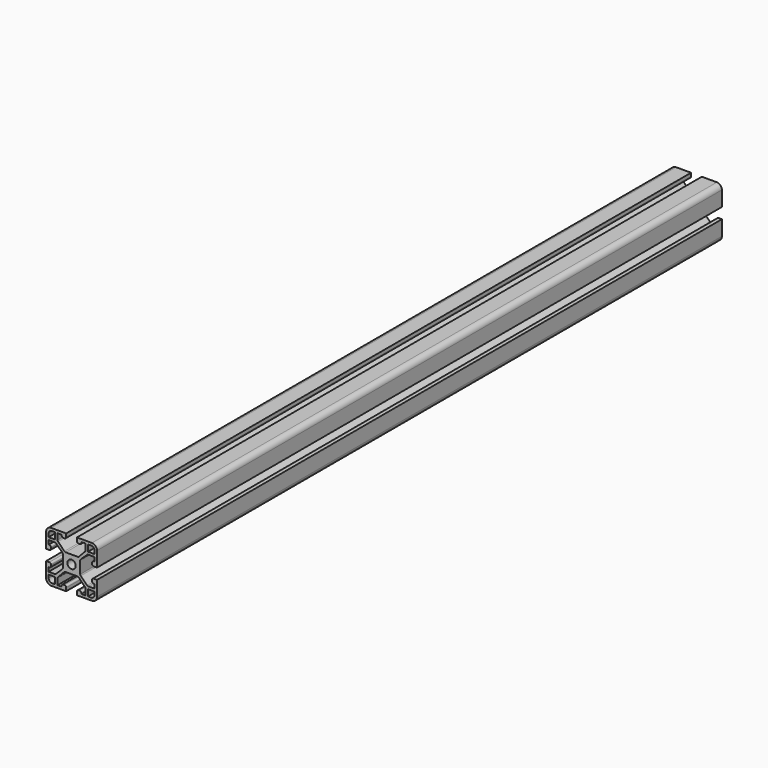
from build123d import *

# Parameters (mm, degrees)
F0_R     = 2.45
F1_DEPTH = 460


# Not quite as in the source:
# - ends of sketch curves that miss each other by under 0.0002 mm in the source are joined


with BuildPart() as f1:
    # F0 (on Front) → F1 (new body)
    with BuildSketch(Plane.XZ):
        with BuildLine():
            Line((-3.1749674082, 15), (-12, 15))
            ThreePointArc((-12, 15), (-14.1213203436, 14.1213203436), (-15, 12))
            Line((-15, 12), (-15, 3.175))
            Line((-15, 3.175), (-13.0855346263, 3.175))
            ThreePointArc((-13.0855346263, 3.175), (-12.3835980145, 3.4627605788), (-12.0856407741, 4.1604300138))
            Line((-12.0856407741, 4.1604300138), (-12.0761692778, 4.8104300138))
            ThreePointArc((-12.0761692778, 4.8104300138), (-12.3638237087, 5.5269366118), (-13.0760631299, 5.825))
            Line((-13.0760631299, 5.825), (-13.5, 5.825))
            Line((-13.5, 5.825), (-13.5, 8.225))
            Line((-13.5, 8.225), (-9.8968845016, 8.225))
            ThreePointArc((-9.8968845016, 8.225), (-9.5279915195, 8.1544718757), (-9.2111331975, 7.9528359354))
            Line((-9.2111331975, 7.9528359354), (-5.4142486959, 4.3754933338))
            ThreePointArc((-5.4142486959, 4.3754933338), (-5.1819174045, 4.0440465354), (-5.1, 3.6476573984))
            Line((-5.1, 3.6476573984), (-5.1, -3.4999243287))
            ThreePointArc((-5.1, -3.4999243287), (-5.1782354607, -3.8876744211), (-5.4007002683, -4.2147528992))
            Line((-5.4007002683, -4.2147528992), (-9.2084959767, -7.9398285705))
            ThreePointArc((-9.2084959767, -7.9398285705), (-9.5301904718, -8.1509666761), (-9.9077957084, -8.225))
            Line((-9.9077957084, -8.225), (-13.5, -8.225))
            Line((-13.5, -8.225), (-13.5, -5.825))
            Line((-13.5, -5.825), (-13.0760631299, -5.825))
            ThreePointArc((-13.0760631299, -5.825), (-12.3638237087, -5.5269366118), (-12.0761692778, -4.8104300138))
            Line((-12.0761692778, -4.8104300138), (-12.0856407741, -4.1604300138))
            ThreePointArc((-12.0856407741, -4.1604300138), (-12.3835980145, -3.4627605788), (-13.0855346263, -3.175))
            Line((-13.0855346263, -3.175), (-15, -3.175))
            Line((-15, -3.175), (-15, -12))
            ThreePointArc((-15, -12), (-14.1213203436, -14.1213203436), (-12, -15))
            Line((-12, -15), (-3.175, -15))
            Line((-3.175, -15), (-3.175, -13.0855346263))
            ThreePointArc((-3.175, -13.0855346263), (-3.4627605788, -12.3835980145), (-4.1604300138, -12.0856407741))
            Line((-4.1604300138, -12.0856407741), (-4.8104300138, -12.0761692778))
            ThreePointArc((-4.8104300138, -12.0761692778), (-5.5269366118, -12.3638237087), (-5.825, -13.0760631299))
            Line((-5.825, -13.0760631299), (-5.825, -13.5))
            Line((-5.825, -13.5), (-8.225, -13.5))
            Line((-8.225, -13.5), (-8.225, -9.8968845016))
            ThreePointArc((-8.225, -9.8968845016), (-8.1544718757, -9.5279915195), (-7.9528359354, -9.2111331975))
            Line((-7.9528359354, -9.2111331975), (-4.3754933338, -5.4142486959))
            ThreePointArc((-4.3754933338, -5.4142486959), (-4.0440465354, -5.1819174045), (-3.6476573984, -5.1))
            Line((-3.6476573984, -5.1), (3.4999243287, -5.1))
            ThreePointArc((3.4999243287, -5.1), (3.8876744211, -5.1782354607), (4.2147528992, -5.4007002683))
            Line((4.2147528992, -5.4007002683), (7.9398285705, -9.2084959767))
            ThreePointArc((7.9398285705, -9.2084959767), (8.1509666761, -9.5301904718), (8.225, -9.9077957084))
            Line((8.225, -9.9077957084), (8.225, -13.5))
            Line((8.225, -13.5), (5.825, -13.5))
            Line((5.825, -13.5), (5.825, -13.0760631299))
            ThreePointArc((5.825, -13.0760631299), (5.5269366118, -12.3638237087), (4.8104300138, -12.0761692778))
            Line((4.8104300138, -12.0761692778), (4.1604300138, -12.0856407741))
            ThreePointArc((4.1604300138, -12.0856407741), (3.4627605788, -12.3835980145), (3.175, -13.0855346263))
            Line((3.175, -13.0855346263), (3.175, -15))
            Line((3.175, -15), (12, -15))
            ThreePointArc((12, -15), (14.1213203436, -14.1213203436), (15, -12))
            Line((15, -12), (15, -3.175))
            Line((15, -3.175), (13.0855346263, -3.175))
            ThreePointArc((13.0855346263, -3.175), (12.3835980145, -3.4627605788), (12.0856407741, -4.1604300138))
            Line((12.0856407741, -4.1604300138), (12.0761692778, -4.8104300138))
            ThreePointArc((12.0761692778, -4.8104300138), (12.3638237087, -5.5269366118), (13.0760631299, -5.825))
            Line((13.0760631299, -5.825), (13.5, -5.825))
            Line((13.5, -5.825), (13.5, -8.225))
            Line((13.5, -8.225), (9.9077957084, -8.225))
            ThreePointArc((9.9077957084, -8.225), (9.5301904718, -8.1509666761), (9.2084959767, -7.9398285705))
            Line((9.2084959767, -7.9398285705), (5.4007002683, -4.2147528992))
            ThreePointArc((5.4007002683, -4.2147528992), (5.1782354607, -3.8876744211), (5.1, -3.4999243287))
            Line((5.1, -3.4999243287), (5.1, 3.6476573984))
            ThreePointArc((5.1, 3.6476573984), (5.1819174045, 4.0440465354), (5.4142486959, 4.3754933338))
            Line((5.4142486959, 4.3754933338), (9.2111331975, 7.9528359354))
            ThreePointArc((9.2111331975, 7.9528359354), (9.5279915195, 8.1544718757), (9.8968845016, 8.225))
            Line((9.8968845016, 8.225), (13.5, 8.225))
            Line((13.5, 8.225), (13.5, 5.825))
            Line((13.5, 5.825), (13.0760631299, 5.825))
            ThreePointArc((13.0760631299, 5.825), (12.3638237087, 5.5269366118), (12.0761692778, 4.8104300138))
            Line((12.0761692778, 4.8104300138), (12.0856407741, 4.1604300138))
            ThreePointArc((12.0856407741, 4.1604300138), (12.3835980145, 3.4627605788), (13.0855346263, 3.175))
            Line((13.0855346263, 3.175), (15, 3.175))
            Line((15, 3.175), (15, 12))
            ThreePointArc((15, 12), (14.1213203436, 14.1213203436), (12, 15))
            Line((12, 15), (3.1750325918, 15))
            Line((3.1750325918, 15), (3.1750325918, 13.0854824722))
            ThreePointArc((3.1750325918, 13.0854824722), (3.4627931706, 12.3835458604), (4.1604626057, 12.0855886201))
            Line((4.1604626057, 12.0855886201), (4.8104626057, 12.0761171237))
            ThreePointArc((4.8104626057, 12.0761171237), (5.5269692036, 12.3637715546), (5.8250325918, 13.0760109758))
            Line((5.8250325918, 13.0760109758), (5.8250325918, 13.4999478459))
            Line((5.8250325918, 13.4999478459), (8.2250325918, 13.4999478459))
            Line((8.2250325918, 13.4999478459), (8.2250325918, 9.8968323476))
            ThreePointArc((8.2250325918, 9.8968323476), (8.1545044675, 9.5279393654), (7.9528685272, 9.2110810434))
            Line((7.9528685272, 9.2110810434), (4.3755259256, 5.4141965418))
            ThreePointArc((4.3755259256, 5.4141965418), (4.0440791272, 5.1818652505), (3.6476899902, 5.0999478459))
            Line((3.6476899902, 5.0999478459), (-3.4998917369, 5.0999478459))
            ThreePointArc((-3.4998917369, 5.0999478459), (-3.8876418293, 5.1781833067), (-4.2147203074, 5.4006481142))
            Line((-4.2147203074, 5.4006481142), (-7.9397959787, 9.2084438226))
            ThreePointArc((-7.9397959787, 9.2084438226), (-8.1509340843, 9.5301383177), (-8.2249674082, 9.9077435543))
            Line((-8.2249674082, 9.9077435543), (-8.2249674082, 13.4999478459))
            Line((-8.2249674082, 13.4999478459), (-5.8249674082, 13.4999478459))
            Line((-5.8249674082, 13.4999478459), (-5.8249674082, 13.0760109758))
            ThreePointArc((-5.8249674082, 13.0760109758), (-5.5269040199, 12.3637715546), (-4.810397422, 12.0761171237))
            Line((-4.810397422, 12.0761171237), (-4.160397422, 12.0855886201))
            ThreePointArc((-4.160397422, 12.0855886201), (-3.462727987, 12.3835458604), (-3.1749674082, 13.0854824722))
            Line((-3.1749674082, 13.0854824722), (-3.1749674082, 15))
        make_face()
        with BuildLine():
            Line((-13.5, -11.5), (-13.5, -9.7))
            Line((-13.5, -9.7), (-9.7, -9.7))
            Line((-9.7, -9.7), (-9.7, -13.5))
            Line((-9.7, -13.5), (-11.5, -13.5))
            ThreePointArc((-11.5, -13.5), (-12.9142135624, -12.9142135624), (-13.5, -11.5))
        make_face(mode=Mode.SUBTRACT)
        with BuildLine():
            Line((9.7, -9.7), (13.5, -9.7))
            Line((13.5, -9.7), (13.5, -11.5))
            ThreePointArc((13.5, -11.5), (12.9142135624, -12.9142135624), (11.5, -13.5))
            Line((11.5, -13.5), (9.7, -13.5))
            Line((9.7, -13.5), (9.7, -9.7))
        make_face(mode=Mode.SUBTRACT)
        with BuildLine():
            ThreePointArc((-13.5, 11.5), (-12.9142135624, 12.9142135624), (-11.5, 13.5))
            Line((-11.5, 13.5), (-9.7, 13.5))
            Line((-9.7, 13.5), (-9.7, 9.7))
            Line((-9.7, 9.7), (-13.5, 9.7))
            Line((-13.5, 9.7), (-13.5, 11.5))
        make_face(mode=Mode.SUBTRACT)
        Circle(F0_R, mode=Mode.SUBTRACT)
        with BuildLine():
            Line((9.7, 13.5), (11.5, 13.5))
            ThreePointArc((11.5, 13.5), (12.9142135624, 12.9142135624), (13.5, 11.5))
            Line((13.5, 11.5), (13.5, 9.7))
            Line((13.5, 9.7), (9.7, 9.7))
            Line((9.7, 9.7), (9.7, 13.5))
        make_face(mode=Mode.SUBTRACT)
    extrude(amount=F1_DEPTH)


solid = f1.part
